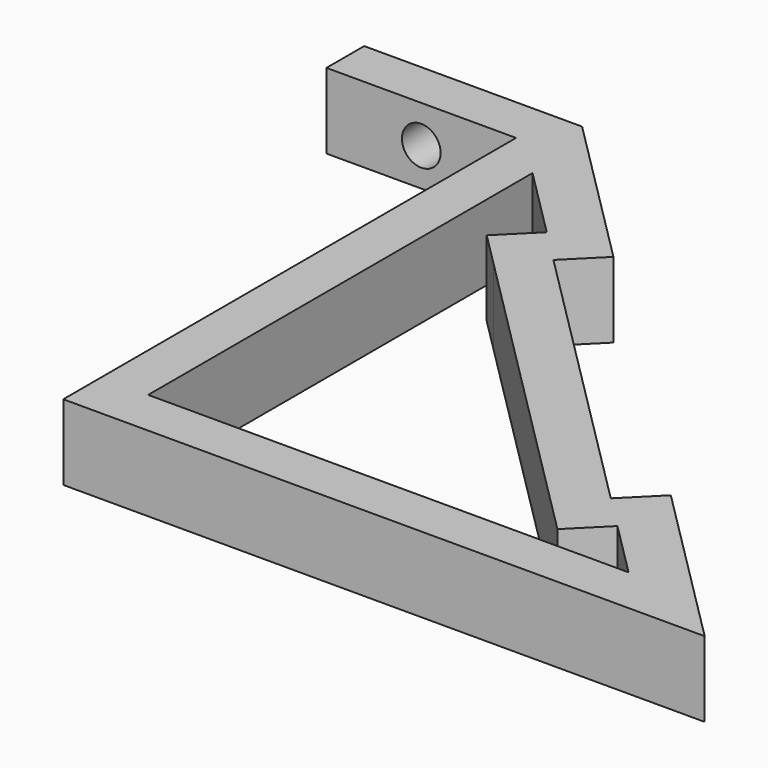
from build123d import *

# Parameters (mm, degrees)
F1_DEPTH    = 8
F3_D        = 4.1
F3_DEPTH    = 7
F3_TIP      = 1.231764269
F4_W        = 43
F4_H        = 8
F5_DEPTH    = 5
F6_T        = 5
F6_T3_DEPTH = 18
F7_D        = 2.8
F7_DEPTH    = 7
F7_TIP      = 0.8412048666


# Not quite as in the source:
# - a shell that OpenCascade refuses in one call is made with other operations: the cavity is built on its own and cut out


with BuildPart() as f1:
    # F0 (on Top) → F1 (new body)
    with BuildSketch(Plane.XY):
        Polygon((22.2267507434, 11.7376726019), (-0.8732492566, 11.7376726019), (-0.8732492566, 6.7376726019), (19.2267507434, 6.7376726019), (19.2267507434, -53.2623273981), (87.2267507434, -53.2623273981), align=None)
    extrude(amount=F1_DEPTH)

    # F3
    with Locations(Plane.XZ.offset(-6.7376726019)):
        with Locations((9.1767507434, 4)):
            Hole(F3_D / 2, depth=F3_DEPTH)
            with Locations((0, 0, -(F3_DEPTH + F3_TIP / 2))):  # 118° drill point
                Cone(0, F3_D / 2, F3_TIP, mode=Mode.SUBTRACT)

    # F4 (on face) → F5 (cut)
    with BuildSketch(Plane(origin=(16.9822116726, 16.9822116726, 0), x_dir=(-0.7071067812, 0.7071067812, 0), z_dir=(0.7071067812, 0.7071067812, 0))):
        with Locations((-52.4168982823, 4)):
            Rectangle(F4_W, F4_H)
    extrude(amount=-F5_DEPTH, mode=Mode.SUBTRACT)

    # F6: shell of thickness 5, made by hand


with BuildPart() as f6_core1:
    # F6_t2: copy of F1
    add(f1.part)

    # the walls: a layer under each face that stays
    f6_faces = [f6_core1.faces().sort_by_distance(p)[0] for p in [
        (18.3767507434, 11.7376726019, 6.6666666667),
        (30.5352554223, 3.4291679229, 4),
        (-0.8732492566, 9.2376726019, 4),
        (7.1267507434, 9.2376726019, 4),
        (37.0759931483, -6.647103709, 4),
        (50.5110219908, -23.6176664575, 4),
        (67.4815847393, -37.0526953, 4),
        (78.2380512178, -44.2736278726, 4),
        (53.2267507434, -53.2623273981, 4),
        (19.2267507434, -23.2623273981, 4),
        (2.4767507434, 6.7376726019, 6.6666666667),
    ]]
    thicken(f6_faces, amount=-F6_T, mode=Mode.SUBTRACT)

    # F6_s4 → F6_t3 (cut)
    with BuildSketch(Plane.XY.offset(-5)):
        Polygon((35.3789368734, -8.414870662), (31.7726922894, -4.879336756), (28.2371583834, -8.414870662), (31.7726922894, -11.9504045679), align=None)
        Polygon((65.7138177863, -38.7497515749), (62.1782838804, -42.3559961589), (65.7138177863, -45.8915300648), (69.2493516923, -42.3559961589), align=None)
        Polygon((19.1767507434, 6.6876726019), (24.2267507434, 6.7376726019), (24.2267507434, 11.7376726019), (19.2267507434, 11.7376726019), align=None)
    extrude(amount=F6_T3_DEPTH, mode=Mode.SUBTRACT)


with BuildPart() as f1_1:
    add(f1.part)

    # what is left inside the walls is the cavity
    f6_cavity = [f6_core1.part.solids().sort_by_distance(p)[0] for p in [
        (49.691217, -31.286017, 0.05),
    ]]
    add(f6_cavity, mode=Mode.SUBTRACT)

    # F7
    with Locations(Plane(origin=(16.9822116726, 16.9822116726, 0), x_dir=(-0.7071067812, 0.7071067812, 0), z_dir=(0.7071067812, 0.7071067812, 0))):
        with Locations((-27.4168982823, 4), (-77.4168982823, 4)):
            Hole(F7_D / 2, depth=F7_DEPTH)
            with Locations((0, 0, -(F7_DEPTH + F7_TIP / 2))):  # 118° drill point
                Cone(0, F7_D / 2, F7_TIP, mode=Mode.SUBTRACT)


solid = f1_1.part
